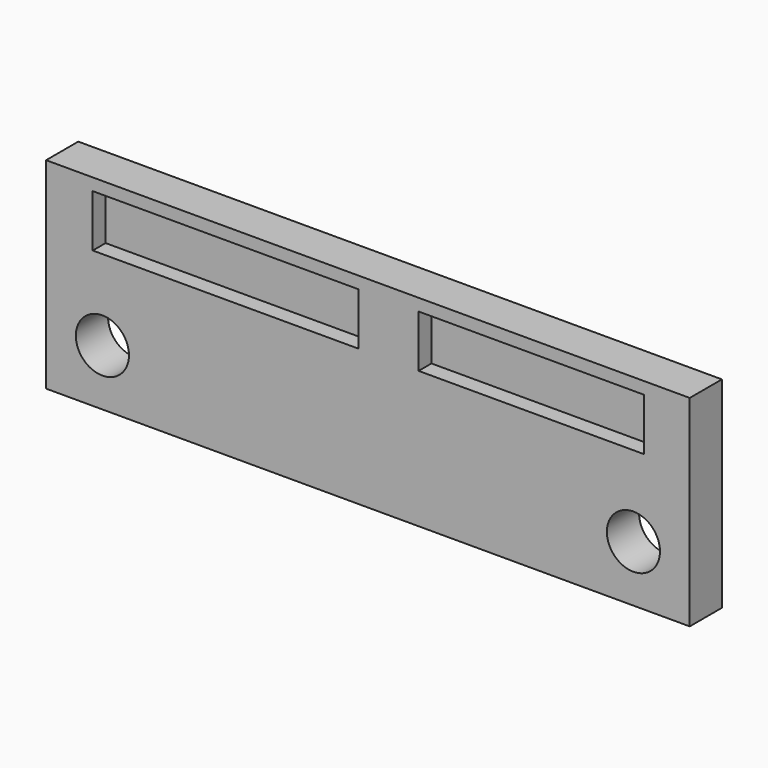
from build123d import *

# Parameters (mm, degrees)
F0_R     = 3.3
F1_DEPTH = 5
F2_W     = 33
F2_H     = 6.5
F2_W_2   = 28
F3_DEPTH = 2


# Not quite as in the source:
# - a feature names something its author has since deleted; it is built from what else it names


with BuildPart() as f1:
    # F0 (on Front) → F1 (new body)
    with BuildSketch(Plane.XZ):
        Polygon((0, 17), (0, 0), (80, 0), (80, 17), (80, 23), (80, 25), (0, 25), (0, 23), align=None)
        with Locations((7, 7)):
            Circle(F0_R, mode=Mode.SUBTRACT)
        with Locations((73, 7)):
            Circle(F0_R, mode=Mode.SUBTRACT)
    extrude(amount=F1_DEPTH)

    # F2 (on face) → F3 (cut)
    with BuildSketch(Plane.XZ.offset(5)):
        with Locations((22.3, 20.25)):
            Rectangle(F2_W, F2_H)
        with Locations((60.3, 20.25)):
            Rectangle(F2_W_2, F2_H)
    extrude(amount=-F3_DEPTH, mode=Mode.SUBTRACT)


solid = f1.part
